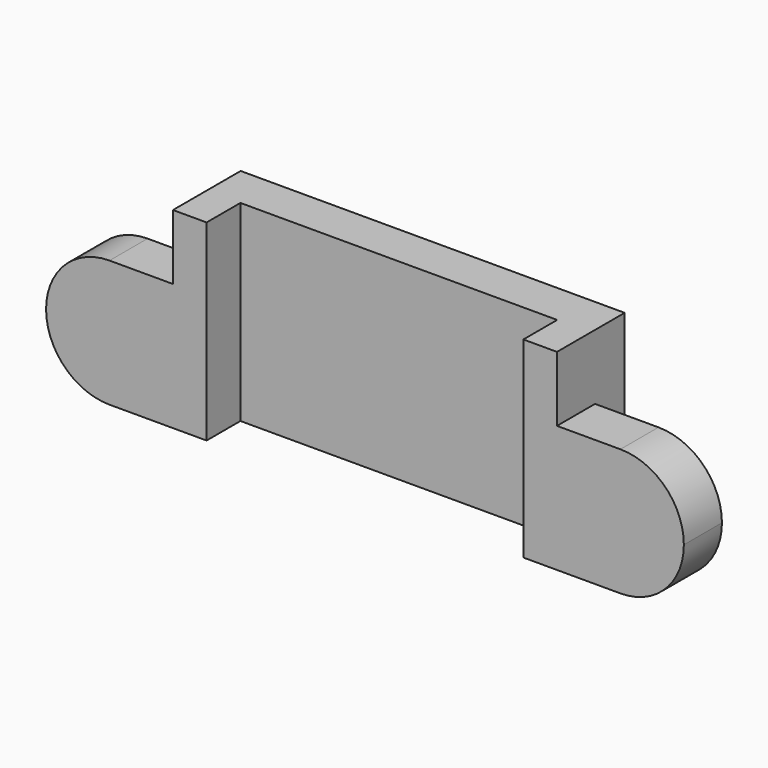
from build123d import *

# Parameters (mm, degrees)
F1_DEPTH = 18.16
F2_W     = 12
F2_H     = 4.5
F3_DEPTH = 12
F4_R     = 5.99999


# Not quite as in the source:
# - a fillet or chamfer is up to 0.001 mm smaller than in the source, because OpenCascade refuses the exact size


with BuildPart() as f1:
    # F0 (on Top) → F1 (new body)
    with BuildSketch(Plane.XY):
        Polygon((18.16, 0), (-18.16, 0), (-18.16, -8), (-14.98, -8), (-14.98, -4), (14.98, -4), (14.98, -8), (18.16, -8), align=None)
    extrude(amount=F1_DEPTH)

    # F2 (on face) → F3 (join)
    with BuildSketch(Plane(origin=(0, 0, 0), x_dir=(1, 0, 0), z_dir=(0, 0, -1))):
        with Locations((-24.16, 5.75)):
            Rectangle(F2_W, F2_H)
        with Locations((24.16, 5.75)):
            Rectangle(F2_W, F2_H)
    extrude(amount=-F3_DEPTH)

    # F4 (radius 6 in the source; OpenCascade refuses exactly that, so slightly less here)
    f4_edges = [f1.edges().sort_by_distance(p)[0] for p in [
        (-30.16, -5.75, 12),
        (-30.16, -5.75, 0),
        (30.16, -5.75, 0),
        (30.16, -5.75, 12),
    ]]
    fillet(f4_edges, radius=F4_R)


solid = f1.part
